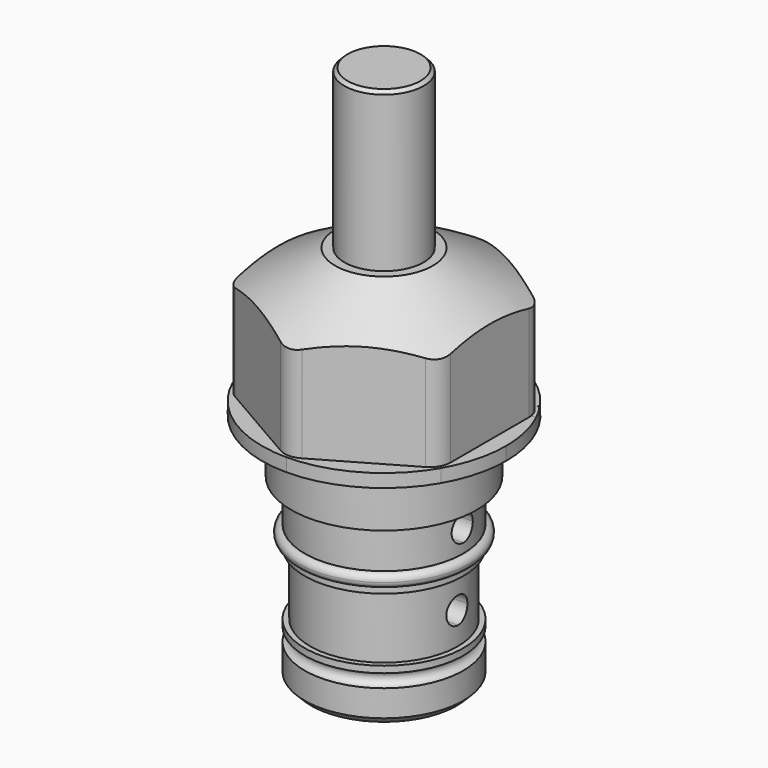
from build123d import *

# Parameters (mm, degrees)
F0_R     = 7.9375
F1_DEPTH = 35.56
F2_DEPTH = 3.175
F3_R     = 5.08
F7_SIZE  = 1.5875
F9_DEPTH = 29.3303937748
F10_W    = 9.525
F10_H    = 37.465
F10_W_2  = 3.175
F10_W_3  = 12.7
F10_H_2  = 22.606
F13_SIZE = 0.79375


with BuildPart() as f1:
    # F0 (on Top) → F1 (new body)
    with BuildSketch(Plane.XY):
        Polygon((25.4, -14.6646968374), (25.4, 14.6646968374), (0, 29.3293936748), (-25.4, 14.6646968374), (-25.4, -14.6646968374), (0, -29.3293936748), align=None)
        Circle(F0_R, mode=Mode.SUBTRACT)
        Circle(F0_R)
    extrude(amount=F1_DEPTH)

    # F0 (on Top) → F2 (join)
    with BuildSketch(Plane.XY):
        with BuildLine():
            ThreePointArc((-25.4, -14.6646968374), (-14.6646968374, -25.4), (0, -29.3293936748))
            Line((0, -29.3293936748), (-25.4, -14.6646968374))
        make_face()
        with BuildLine():
            ThreePointArc((0, -29.3293936748), (14.6646968374, -25.4), (25.4, -14.6646968374))
            Line((25.4, -14.6646968374), (0, -29.3293936748))
        make_face()
        with BuildLine():
            ThreePointArc((25.4, -14.6646968374), (28.3300188199, -7.5910056644), (29.3293936748, 0))
            ThreePointArc((29.3293936748, 0), (28.3300188199, 7.5910056644), (25.4, 14.6646968374))
            Line((25.4, 14.6646968374), (25.4, -14.6646968374))
        make_face()
        Polygon((25.4, -14.6646968374), (25.4, 14.6646968374), (0, 29.3293936748), (-25.4, 14.6646968374), (-25.4, -14.6646968374), (0, -29.3293936748), align=None)
        Circle(F0_R, mode=Mode.SUBTRACT)
        with BuildLine():
            Line((0, 29.3293936748), (25.4, 14.6646968374))
            ThreePointArc((25.4, 14.6646968374), (14.6646968374, 25.4), (0, 29.3293936748))
        make_face()
        with BuildLine():
            Line((-25.4, 14.6646968374), (0, 29.3293936748))
            ThreePointArc((0, 29.3293936748), (-14.6646968374, 25.4), (-25.4, 14.6646968374))
        make_face()
        with BuildLine():
            Line((-25.4, -14.6646968374), (-25.4, 14.6646968374))
            ThreePointArc((-25.4, 14.6646968374), (-29.3293936748, 0), (-25.4, -14.6646968374))
        make_face()
    extrude(amount=F2_DEPTH)

    # F3 (call 1 of 6: OpenCascade refuses the feature's edges together)
    f3_edges = [f1.edges().sort_by_distance(p)[0] for p in [
        (0, -29.329394, 19.3675),
    ]]
    fillet(f3_edges, radius=F3_R)

    # F3#2 (call 2 of 6)
    f3_2_edges = [f1.edges().sort_by_distance(p)[0] for p in [
        (25.4, -14.664697, 19.3675),
    ]]
    fillet(f3_2_edges, radius=F3_R)

    # F3#3 (call 3 of 6)
    f3_3_edges = [f1.edges().sort_by_distance(p)[0] for p in [
        (25.4, 14.664697, 19.3675),
    ]]
    fillet(f3_3_edges, radius=F3_R)

    # F3#4 (call 4 of 6)
    f3_4_edges = [f1.edges().sort_by_distance(p)[0] for p in [
        (0, 29.329394, 19.3675),
    ]]
    fillet(f3_4_edges, radius=F3_R)

    # F3#5 (call 5 of 6)
    f3_5_edges = [f1.edges().sort_by_distance(p)[0] for p in [
        (-25.4, 14.664697, 19.3675),
    ]]
    fillet(f3_5_edges, radius=F3_R)

    # F3#6 (call 6 of 6)
    f3_6_edges = [f1.edges().sort_by_distance(p)[0] for p in [
        (-25.4, -14.664697, 19.3675),
    ]]
    fillet(f3_6_edges, radius=F3_R)

    # F4 (on Right) → F5 (revolve, cut)
    with BuildSketch(Plane.YZ):
        Polygon((35.3962906179, 35.56), (11.7317574699, 35.56), (35.3962906179, 21.8972754168), align=None)
    revolve(axis=Axis((0, 0, 25.9955581278), (0, 0, -1)), mode=Mode.SUBTRACT)

    # F4 (on Right) → F6 (revolve)
    with BuildSketch(Plane.YZ):
        with BuildLine():
            Line((17.78, -27.686), (0, -27.686))
            Line((0, -27.686), (0, -32.131))
            ThreePointArc((0, -32.131), (2.2450640303, -33.0609359697), (3.175, -35.306))
            ThreePointArc((3.175, -35.306), (2.2450640303, -37.5510640303), (0, -38.481))
            Line((0, -38.481), (0, -42.926))
            Line((0, -42.926), (17.78, -42.926))
            Line((17.78, -42.926), (17.78, -27.686))
        make_face()
        with BuildLine():
            Line((19.05, -12.7), (0, -12.7))
            Line((0, -12.7), (0, -14.2875))
            ThreePointArc((0, -14.2875), (2.2450640303, -15.2174359697), (3.175, -17.4625))
            ThreePointArc((3.175, -17.4625), (2.2450640303, -19.7075640303), (0, -20.6375))
            Line((0, -20.6375), (0, -27.686))
            Line((0, -27.686), (17.78, -27.686))
            Line((17.78, -27.686), (19.05, -27.686))
            Line((19.05, -27.686), (19.05, -26.0985))
            ThreePointArc((19.05, -26.0985), (17.4625, -24.511), (19.05, -22.9235))
            Line((19.05, -22.9235), (19.05, -12.7))
        make_face()
        Polygon((22.225, 0), (0, 0), (0, -12.7), (19.05, -12.7), (22.225, -12.7), align=None)
        with BuildLine():
            Line((19.05, -42.926), (17.78, -42.926))
            Line((17.78, -42.926), (0, -42.926))
            Line((0, -42.926), (0, -55.626))
            Line((0, -55.626), (19.05, -55.626))
            Line((19.05, -55.626), (19.05, -47.6885))
            ThreePointArc((19.05, -47.6885), (17.4625, -46.101), (19.05, -44.5135))
            Line((19.05, -44.5135), (19.05, -42.926))
        make_face()
    revolve(axis=Axis((0, 0, 25.9955581278), (0, 0, -1)))

    # F7
    f7_edges = [f1.edges().sort_by_distance(p)[0] for p in [
        (0, -19.05, -55.626),
    ]]
    chamfer(f7_edges, length=F7_SIZE)


with BuildPart() as f8:
    # F4 (on Right) → F8 (revolve)
    with BuildSketch(Plane.YZ):
        with BuildLine():
            Line((0, -20.6375), (0, -14.2875))
            ThreePointArc((0, -14.2875), (-3.175, -17.4625), (0, -20.6375))
        make_face()
    revolve(axis=Axis((0, 0, 25.9955581278), (0, 0, -1)))


with BuildPart() as f8b:
    # F4 (on Right) → F8, piece 2 (revolve)
    with BuildSketch(Plane.YZ):
        with BuildLine():
            ThreePointArc((20.6375, -24.511), (20.1725320151, -23.3884679849), (19.05, -22.9235))
            Line((19.05, -22.9235), (19.05, -26.0985))
            ThreePointArc((19.05, -26.0985), (20.1725320151, -25.6335320151), (20.6375, -24.511))
        make_face()
        with BuildLine():
            Line((19.05, -26.0985), (19.05, -22.9235))
            ThreePointArc((19.05, -22.9235), (17.4625, -24.511), (19.05, -26.0985))
        make_face()
    revolve(axis=Axis((0, 0, 25.9955581278), (0, 0, -1)))


with BuildPart() as f9_tool:
    # F4 (on Right) → F9 (new body, through all)
    with BuildSketch(Plane.YZ):
        with BuildLine():
            Line((0, -20.6375), (0, -14.2875))
            ThreePointArc((0, -14.2875), (-3.175, -17.4625), (0, -20.6375))
        make_face()
        with BuildLine():
            ThreePointArc((3.175, -17.4625), (2.2450640303, -15.2174359697), (0, -14.2875))
            Line((0, -14.2875), (0, -20.6375))
            ThreePointArc((0, -20.6375), (2.2450640303, -19.7075640303), (3.175, -17.4625))
        make_face()
        with BuildLine():
            Line((0, -38.481), (0, -32.131))
            ThreePointArc((0, -32.131), (-3.175, -35.306), (0, -38.481))
        make_face()
        with BuildLine():
            ThreePointArc((3.175, -35.306), (2.2450640303, -33.0609359697), (0, -32.131))
            Line((0, -32.131), (0, -38.481))
            ThreePointArc((0, -38.481), (2.2450640303, -37.5510640303), (3.175, -35.306))
        make_face()
    extrude(amount=F9_DEPTH)


with BuildPart() as f1_1:
    add(f1.part)

    # F9: cut by f9_tool
    add(f9_tool.part, mode=Mode.SUBTRACT)


with BuildPart() as f8_1:
    add(f8.part)

    # F9: cut by f9_tool
    add(f9_tool.part, mode=Mode.SUBTRACT)


with BuildPart() as f11_tool:
    # F10 (on Right) → F11 (revolve)
    with BuildSketch(Plane.YZ):
        Polygon((9.525, 73.66), (0, 73.66), (0, 15.875), (9.525, 15.875), (9.525, 21.374261314), align=None)
        Polygon((9.525, 21.374261314), (9.525, 15.875), (12.7, 15.875), align=None)
        with Locations((4.7625, -2.8575)):
            Rectangle(F10_W, F10_H)
        with Locations((11.1125, -2.8575)):
            Rectangle(F10_W_2, F10_H)
        with Locations((6.35, -39.243)):
            Rectangle(F10_W_3, F10_H_2)
        Polygon((9.525, -21.59), (0, -21.59), (0, -27.94), (12.7, -27.94), (12.7, -21.59), align=None)
    revolve(axis=Axis((0, 0, 11.557), (0, 0, -1)))


with BuildPart() as f1_2:
    add(f1_1.part)

    # F11: cut by f11_tool
    add(f11_tool.part, mode=Mode.SUBTRACT)


with BuildPart() as f8_2:
    add(f8_1.part)

    # F11: cut by f11_tool
    add(f11_tool.part, mode=Mode.SUBTRACT)


with BuildPart() as f12:
    # F10 (on Right) → F12 (revolve)
    with BuildSketch(Plane.YZ):
        Polygon((9.525, 73.66), (0, 73.66), (0, 15.875), (9.525, 15.875), (9.525, 21.374261314), align=None)
        with Locations((4.7625, -2.8575)):
            Rectangle(F10_W, F10_H)
        Polygon((9.525, -21.59), (0, -21.59), (0, -27.94), (12.7, -27.94), (12.7, -21.59), align=None)
    revolve(axis=Axis((0, 0, 11.557), (0, 0, -1)))

    # F13
    f13_edges = [f12.edges().sort_by_distance(p)[0] for p in [
        (0, -9.525, 73.66),
    ]]
    chamfer(f13_edges, length=F13_SIZE)


solid = Compound([f8b.part, f1_2.part, f12.part])
